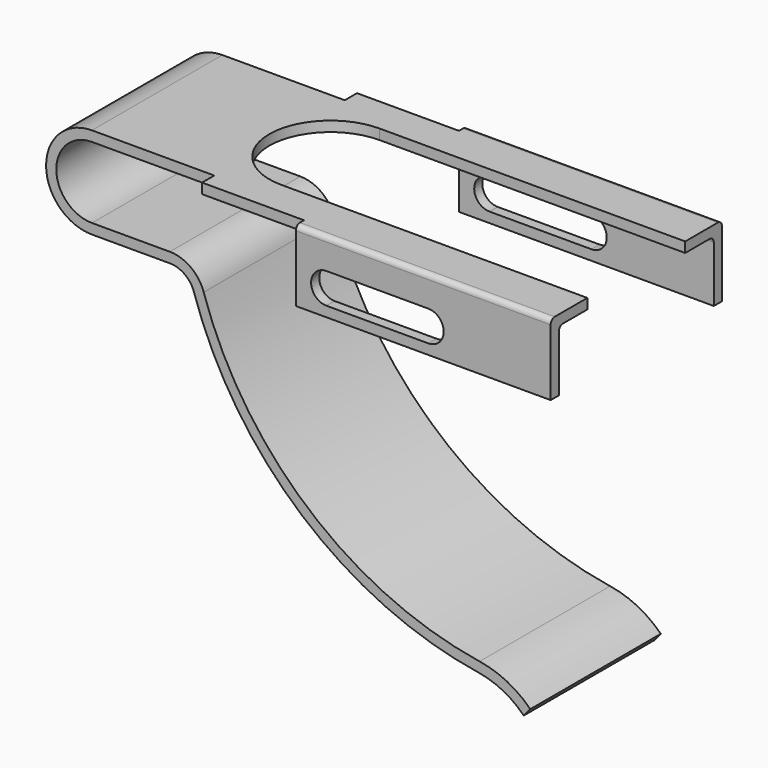
from build123d import *

# Parameters (mm, degrees)
F1_DEPTH  = 16
F2_W      = 70
F2_H      = 3
F3_DEPTH  = 2
F4_W      = 50
F4_H      = 14
F5_DEPTH  = 2
F6_R      = 1
F9_DEPTH  = 2
F11_DEPTH = 42.001


with BuildPart() as f1:
    # F0 (on Front) → F1 (new body)
    with BuildSketch(Plane.XZ):
        with BuildLine():
            Line((94, 9), (0, 9))
            ThreePointArc((0, 9), (-9, 0), (0, -9))
            Line((0, -9), (15.2698143006, -9))
            ThreePointArc((15.2698143006, -9), (18.2087071496, -9.9548907528), (20.0250713566, -12.4548364712))
            ThreePointArc((20.0250713566, -12.4548364712), (41.226339877, -44.1268775333), (75.8783002618, -59.9967739854))
            ThreePointArc((75.8783002618, -59.9967739854), (80.6596281551, -61.5636317865), (84.7179401809, -64.5378952739))
            Line((84.7179401809, -64.5378952739), (86.0083877193, -62.9999997839))
            ThreePointArc((86.0083877193, -62.9999997839), (81.4277187811, -59.7105770288), (76.0540091245, -57.9999997839))
            ThreePointArc((76.0540091245, -57.9999997839), (42.4723911749, -42.5610388699), (21.9271739736, -11.8367711264))
            ThreePointArc((21.9271739736, -11.8367711264), (19.3842641622, -8.3368472287), (15.2698143006, -7.0000002161))
            Line((15.2698143006, -7.0000002161), (0, -7.0000002161))
            ThreePointArc((0, -7.0000002161), (-7.0000002161, 0), (0, 7.0000002161))
            Line((0, 7.0000002161), (94, 7.0000002161))
            Line((94, 7.0000002161), (94, 9))
        make_face()
    extrude(amount=F1_DEPTH)

    # F2 (on face) → F3 (join)
    with BuildSketch(Plane.XY.offset(9)):
        with Locations((59, -17.5)):
            Rectangle(F2_W, F2_H)
    extrude(amount=-F3_DEPTH)

    # F4 (on face) → F5 (join)
    with BuildSketch(Plane.XZ.offset(19)):
        with Locations((69, 2)):
            Rectangle(F4_W, F4_H)
    extrude(amount=F5_DEPTH)

    # F6
    f6_edges = [f1.edges().sort_by_distance(p)[0] for p in [
        (69, -21, 9),
        (69, -19, 7),
    ]]
    fillet(f6_edges, radius=F6_R)

    # F7: F1 across plane


with BuildPart() as f1_1:
    add(f1.part)
    add(f1.part.mirror(Plane.XZ))

    # F8 (on face) → F9 (cut)
    with BuildSketch(Plane.XY.offset(9)):
        with BuildLine():
            Line((94, 12), (34, 12))
            ThreePointArc((34, 12), (22, 0), (34, -12))
            Line((34, -12), (94, -12))
            Line((94, -12), (94, 12))
        make_face()
    extrude(amount=-F9_DEPTH, mode=Mode.SUBTRACT)

    # F10 (on face) → F11 (cut, through all)
    with BuildSketch(Plane.XZ.offset(21)):
        with BuildLine():
            ThreePointArc((50, 3), (47, 0), (50, -3))
            Line((50, -3), (70, -3))
            ThreePointArc((70, -3), (73, 0), (70, 3))
            Line((70, 3), (50, 3))
        make_face()
    extrude(amount=-F11_DEPTH, mode=Mode.SUBTRACT)


solid = f1_1.part
